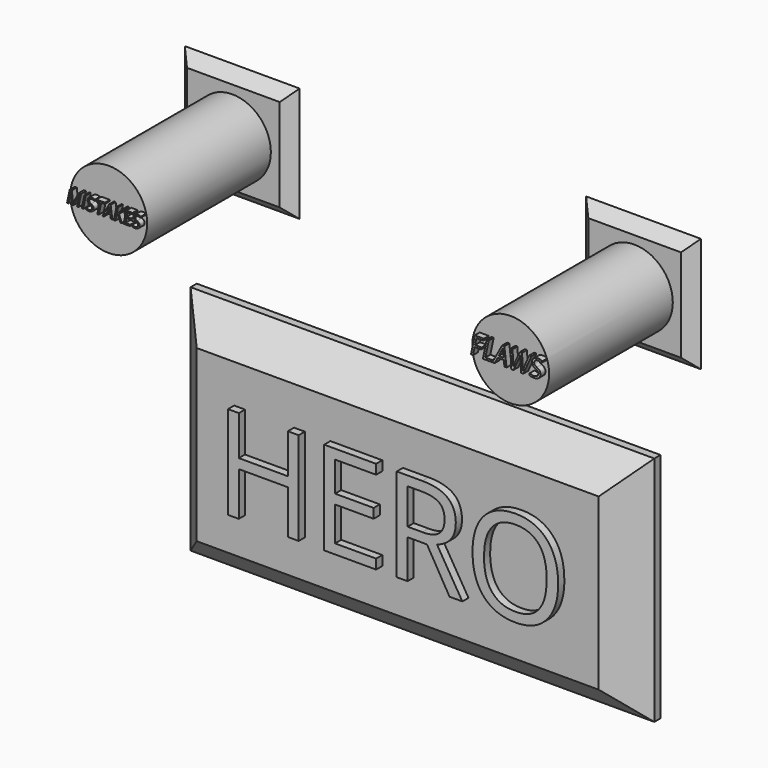
from build123d import *

# Parameters (mm, degrees)
F0_W          = 25.4
F0_H          = 25.4000019861
F1_DEPTH      = 1.8142857143
F0_H_2        = 25.4
F2_T1_DEPTH   = 51.5283011438
F2_T3_DEPTH   = 51.5282991577
F2_2_T1_DEPTH = 51.5282991577
F2_2_T3_DEPTH = 51.5282991577
F3_R          = 6.3199469448
F4_DEPTH      = 25.4
F5_TEXT_SIZE  = 2.8823545125
F6_TEXT_SIZE  = 4.1462706933
F7_DEPTH      = 1.016
F8_W          = 76.2
F8_H          = 38.1
F9_DEPTH      = 6.35
F10_SIZE      = 5.08
F11_TEXT_SIZE = 21.4291658873
F12_DEPTH     = 1.27


# Not quite as in the source:
# - a fillet or chamfer that OpenCascade refuses, or shapes differently, is made with other operations: its cross-section is extruded or revolved along the edge and cut away or added
# - Text() gives the source's letters only with a copy of the font that has no kerning and outlines rounded to 1/6400 em; it was checked with that copy


with BuildPart() as f1:
    # F0 (on Front) → F1 (new body)
    with BuildSketch(Plane.XZ):
        with Locations((-95.6447347999, 18.7335992232)):
            Rectangle(F0_W, F0_H)
    extrude(amount=F1_DEPTH)

    # F2: chamfer of 5.08 on 4 edges, made by hand

    # F2_s2 → F2_t1 (cut)
    with BuildSketch(Plane.XY.offset(-7.0305513487)):
        Polygon((-82.9447347999, 3.2657142857), (-88.0247347999, -1.8142857143), (-82.9447347999, -1.8142857143), align=None)
        Polygon((-108.3447347999, 3.2657142857), (-103.2647347999, -1.8142857143), (-108.3447347999, -1.8142857143), align=None)
    extrude(amount=F2_T1_DEPTH, mode=Mode.SUBTRACT)

    # F2_s4 → F2_t3 (cut)
    with BuildSketch(Plane.YZ.offset(-121.4088843787)):
        Polygon((3.2657142857, 31.4336002162), (-1.8142857143, 26.3536002162), (-1.8142857143, 31.4336002162), align=None)
        Polygon((3.2657142857, 6.0335982302), (-1.8142857143, 11.1135982302), (-1.8142857143, 6.0335982302), align=None)
    extrude(amount=F2_T3_DEPTH, mode=Mode.SUBTRACT)

    # F3 (on face) → F4 (join)
    with BuildSketch(Plane.XZ.offset(1.8142857143)):
        with Locations((-95.804207027, 18.6266154051)):
            Circle(F3_R)
    extrude(amount=F4_DEPTH)



with BuildPart() as f1b:
    # F0 (on Front) → F1, piece 2 (new body)
    with BuildSketch(Plane.XZ):
        with Locations((-29.7082279205, 18.4341400534)):
            Rectangle(F0_W, F0_H_2)
    extrude(amount=F1_DEPTH)

    # F2#2: chamfer of 5.08 on 4 edges, made by hand

    # F2_2_s2 → F2_2_t1 (cut)
    with BuildSketch(Plane.YZ.offset(-55.4723774994)):
        Polygon((3.2657142857, 31.1341400534), (-1.8142857143, 26.0541400534), (-1.8142857143, 31.1341400534), align=None)
        Polygon((3.2657142857, 5.7341400534), (-1.8142857143, 10.8141400534), (-1.8142857143, 5.7341400534), align=None)
    extrude(amount=F2_2_T1_DEPTH, mode=Mode.SUBTRACT)

    # F2_2_s4 → F2_2_t3 (cut)
    with BuildSketch(Plane.XY.offset(-7.3300095255)):
        Polygon((-42.4082279205, 3.2657142857), (-37.3282279205, -1.8142857143), (-42.4082279205, -1.8142857143), align=None)
        Polygon((-17.0082279205, 3.2657142857), (-22.0882279205, -1.8142857143), (-17.0082279205, -1.8142857143), align=None)
    extrude(amount=F2_2_T3_DEPTH, mode=Mode.SUBTRACT)

    # F3 (on face) → F4, piece 2 (join)
    with BuildSketch(Plane.XZ.offset(1.8142857143)):
        with Locations((-29.7638233751, 18.3744449168)):
            Circle(F3_R)
    extrude(amount=F4_DEPTH)


with BuildPart() as f1_1:
    add(f1.part)

    add(f1b.part)  # F7 merges F1b
    # F5 (on face) + F6 (on face) → F7 (join)
    with BuildSketch(Plane.XZ.offset(27.2142857143)):
        with Locations((-101.9528493767, 18.0128011309)):
            Text('MISTAKES', F5_TEXT_SIZE, font='Open Sans', font_style=FontStyle.ITALIC, text_align=(TextAlign.LEFT, TextAlign.BOTTOM))
    with BuildSketch(Plane.XZ.offset(27.2142857143)):
        with Locations((-35.6522686549, 17.6843296979)):
            Text('FLAWS', F6_TEXT_SIZE, font='Open Sans', font_style=FontStyle.ITALIC, text_align=(TextAlign.LEFT, TextAlign.BOTTOM))
    extrude(amount=F7_DEPTH)


with BuildPart() as f9:
    # F8 (on Front) → F9 (new body)
    with BuildSketch(Plane.XZ):
        with Locations((-65.0153663009, -24.601847123)):
            Rectangle(F8_W, F8_H)
    extrude(amount=F9_DEPTH)

    # F10
    f10_edges = [f9.edges().sort_by_distance(p)[0] for p in [
        (-65.015366, -6.35, -5.551847),
        (-103.115366, -6.35, -24.601847),
        (-65.015366, -6.35, -43.651847),
        (-26.915366, -6.35, -24.601847),
    ]]
    chamfer(f10_edges, length=F10_SIZE)

    # F11 (on face) → F12 (join)
    with BuildSketch(Plane.XZ.offset(6.35)):
        with Locations((-93.9871966839, -32.250540331)):
            Text('HERO', F11_TEXT_SIZE, font='Open Sans', text_align=(TextAlign.LEFT, TextAlign.BOTTOM))
    extrude(amount=F12_DEPTH)


solid = Compound([f1_1.part, f9.part])
